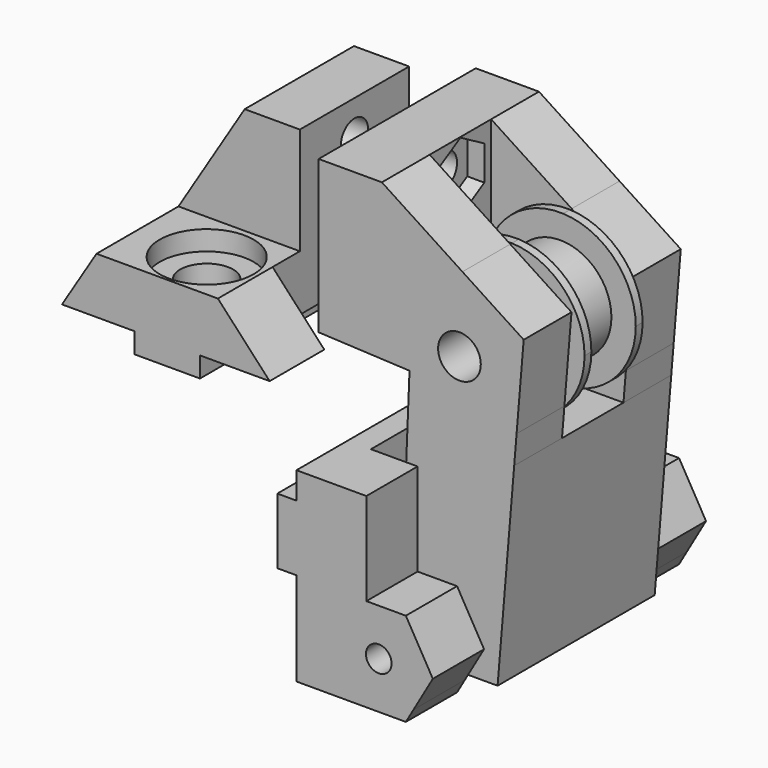
from build123d import *

# Parameters (mm, degrees)
F0_R      = 1.5
F1_DEPTH  = 20
F2_DEPTH  = 12.5
F0_R_2    = 6
F0_R_3    = 2.5
F3_DEPTH  = 4.25
F4_DEPTH  = 3.25
F5_DEPTH  = 11.5
F6_DEPTH  = 4.5
F7_DEPTH  = 20
F0_W      = 6.4631571341
F0_H      = 12.5490699407
F8_DEPTH  = 8
F9_DEPTH  = 5
F10_R     = 2
F11_DEPTH = 25
F12_DEPTH = 2
F13_R     = 3.1
F14_DEPTH = 9.6
F13_R_2   = 5.5
F15_DEPTH = 2.3
F16_DEPTH = 12


# Not quite as in the source:
# - a feature names something its author has since deleted; it is built from what else it names


with BuildPart() as f1:
    # F0 (on Front) → F1 (new body, symmetric)
    with BuildSketch(Plane.XZ):
        Polygon((12.0433680713, 8.4268744104), (9.800856933, 8.4268744104), (9.800856933, 0.7268744104), (12.0433680713, 0.7268744104), (12.0433680713, -4.5145147916), (12.0433680713, -4.9838108923), (12.0433680713, -10.2252000943), (14.7645920515, -10.2252000943), (14.7645920515, 11.5647632629), (12.0433680713, 11.5647632629), align=None)
        Polygon((18.1240398149, 11.5647632629), (14.7645920515, 11.5647632629), (14.7645920515, -10.2252000943), (24.8542597735, -10.2252000943), (25.7545311213, -8.6658843793), (17.3043143004, -8.6658843793), align=None)
        Polygon((20.2310747576, 11.5647632629), (18.1240398149, 11.5647632629), (17.3043143004, -8.6658843793), (25.7545311213, -8.6658843793), (28.0158513552, -4.749162842), (24.8542597735, 0.7268744104), (20.2310747576, 0.7268744104), align=None)
        with Locations((21.6832533479, -4.7491648653)):
            Circle(F0_R, mode=Mode.SUBTRACT)
    extrude(amount=F1_DEPTH, both=True)

    # F0 (on Front) → F2 (cut, symmetric)
    with BuildSketch(Plane.XZ):
        Polygon((20.2310747576, 11.5647632629), (18.1240398149, 11.5647632629), (17.3043143004, -8.6658843793), (25.7545311213, -8.6658843793), (28.0158513552, -4.749162842), (24.8542597735, 0.7268744104), (20.2310747576, 0.7268744104), align=None)
        with Locations((21.6832533479, -4.7491648653)):
            Circle(F0_R, mode=Mode.SUBTRACT)
        Polygon((18.1240398149, 11.5647632629), (14.7645920515, 11.5647632629), (14.7645920515, -10.2252000943), (24.8542597735, -10.2252000943), (25.7545311213, -8.6658843793), (17.3043143004, -8.6658843793), align=None)
    extrude(amount=F2_DEPTH, both=True, mode=Mode.SUBTRACT)


with BuildPart() as f3:
    # F0 (on Front) → F3 (new body, symmetric)
    with BuildSketch(Plane.XZ):
        with BuildLine():
            Line((18.4845160693, 20.4612389207), (18.3568896242, 17.3114459771))
            ThreePointArc((18.3568896242, 17.3114459771), (24.8470334947, 15.0024096492), (31.0266731703, 18.0463659077))
            Line((31.0266731703, 18.0463659077), (31.8562861888, 28.0017219973))
            Line((31.8562861888, 28.0017219973), (24.6849621756, 32.6806183183))
            ThreePointArc((24.6849621756, 32.6806183183), (17.1127643071, 28.953063684), (16.1086398476, 20.5730530528))
            Line((16.1086398476, 20.5730530528), (18.4845160693, 20.4612389207))
        make_face()
        with Locations((24.3345443159, 23.8375584789)):
            Circle(F0_R_2, mode=Mode.SUBTRACT)
        with Locations((24.3345443159, 23.8375584789)):
            Circle(F0_R_2)
        with Locations((24.3345443159, 23.8375584789)):
            Circle(F0_R_3, mode=Mode.SUBTRACT)
        with BuildLine():
            Line((31.8562861888, 28.0017219973), (31.0266731703, 18.0463659077))
            ThreePointArc((31.0266731703, 18.0463659077), (32.6275486075, 20.7474808392), (33.1845443159, 23.8375584789))
            ThreePointArc((33.1845443159, 23.8375584789), (30.7151280689, 29.970310795), (24.6849621756, 32.6806183183))
            Line((24.6849621756, 32.6806183183), (31.8562861888, 28.0017219973))
        make_face()
        with BuildLine():
            ThreePointArc((16.1086398476, 20.5730530528), (17.0479268988, 18.8148394327), (18.3568896242, 17.3114459771))
            Line((18.3568896242, 17.3114459771), (18.4845160693, 20.4612389207))
            Line((18.4845160693, 20.4612389207), (16.1086398476, 20.5730530528))
        make_face()
    extrude(amount=F3_DEPTH, both=True)

    # F0 (on Front) → F4 (cut, symmetric)
    with BuildSketch(Plane.XZ):
        with BuildLine():
            Line((31.8562861888, 28.0017219973), (31.0266731703, 18.0463659077))
            ThreePointArc((31.0266731703, 18.0463659077), (32.6275486075, 20.7474808392), (33.1845443159, 23.8375584789))
            ThreePointArc((33.1845443159, 23.8375584789), (30.7151280689, 29.970310795), (24.6849621756, 32.6806183183))
            Line((24.6849621756, 32.6806183183), (31.8562861888, 28.0017219973))
        make_face()
        with BuildLine():
            Line((18.4845160693, 20.4612389207), (18.3568896242, 17.3114459771))
            ThreePointArc((18.3568896242, 17.3114459771), (24.8470334947, 15.0024096492), (31.0266731703, 18.0463659077))
            Line((31.0266731703, 18.0463659077), (31.8562861888, 28.0017219973))
            Line((31.8562861888, 28.0017219973), (24.6849621756, 32.6806183183))
            ThreePointArc((24.6849621756, 32.6806183183), (17.1127643071, 28.953063684), (16.1086398476, 20.5730530528))
            Line((16.1086398476, 20.5730530528), (18.4845160693, 20.4612389207))
        make_face()
        with Locations((24.3345443159, 23.8375584789)):
            Circle(F0_R_2, mode=Mode.SUBTRACT)
        with BuildLine():
            ThreePointArc((16.1086398476, 20.5730530528), (17.0479268988, 18.8148394327), (18.3568896242, 17.3114459771))
            Line((18.3568896242, 17.3114459771), (18.4845160693, 20.4612389207))
            Line((18.4845160693, 20.4612389207), (16.1086398476, 20.5730530528))
        make_face()
    extrude(amount=F4_DEPTH, both=True, mode=Mode.SUBTRACT)


with BuildPart() as f5:
    # F0 (on Front) → F5 (new body, symmetric)
    with BuildSketch(Plane.XZ):
        with BuildLine():
            Line((18.4845160693, 20.4612389207), (18.3568896242, 17.3114459771))
            ThreePointArc((18.3568896242, 17.3114459771), (24.8470334947, 15.0024096492), (31.0266731703, 18.0463659077))
            Line((31.0266731703, 18.0463659077), (31.8562861888, 28.0017219973))
            Line((31.8562861888, 28.0017219973), (24.6849621756, 32.6806183183))
            ThreePointArc((24.6849621756, 32.6806183183), (17.1127643071, 28.953063684), (16.1086398476, 20.5730530528))
            Line((16.1086398476, 20.5730530528), (18.4845160693, 20.4612389207))
        make_face()
        with Locations((24.3345443159, 23.8375584789)):
            Circle(F0_R_2, mode=Mode.SUBTRACT)
        Polygon((18.2491015751, 14.6512603387), (18.1240398149, 11.5647632629), (20.2310747576, 11.5647632629), (20.2310747576, 0.7268744104), (24.8542597735, 0.7268744104), (28.0158513552, -4.749162842), (25.7545311213, -8.6658843793), (28.8006522836, -8.6658843793), (30.7437477025, 14.6512603387), align=None)
        Polygon((7.8407172114, 20.9621602735), (15.2479996905, 20.6135567336), (15.2479996905, 38.8377197087), (7.8407172114, 38.8377197087), align=None)
        with Locations((24.3345443159, 23.8375584789)):
            Circle(F0_R_2)
        with Locations((24.3345443159, 23.8375584789)):
            Circle(F0_R_3, mode=Mode.SUBTRACT)
        Polygon((20.2310747576, 11.5647632629), (18.1240398149, 11.5647632629), (17.3043143004, -8.6658843793), (25.7545311213, -8.6658843793), (28.0158513552, -4.749162842), (24.8542597735, 0.7268744104), (20.2310747576, 0.7268744104), align=None)
        with Locations((21.6832533479, -4.7491648653)):
            Circle(F0_R, mode=Mode.SUBTRACT)
        with BuildLine():
            Line((15.2479996905, 20.6135567336), (16.1086398476, 20.5730530528))
            ThreePointArc((16.1086398476, 20.5730530528), (17.1127643071, 28.953063684), (24.6849621756, 32.6806183183))
            Line((24.6849621756, 32.6806183183), (15.2479996905, 38.8377197087))
            Line((15.2479996905, 38.8377197087), (15.2479996905, 20.6135567336))
        make_face()
        with BuildLine():
            Line((18.3568896242, 17.3114459771), (18.2491015751, 14.6512603387))
            Line((18.2491015751, 14.6512603387), (30.7437477025, 14.6512603387))
            Line((30.7437477025, 14.6512603387), (31.0266731703, 18.0463659077))
            ThreePointArc((31.0266731703, 18.0463659077), (24.8470334947, 15.0024096492), (18.3568896242, 17.3114459771))
        make_face()
    extrude(amount=F5_DEPTH, both=True)

    # F0 (on Front) → F6 (cut, symmetric)
    with BuildSketch(Plane.XZ):
        with BuildLine():
            Line((18.4845160693, 20.4612389207), (18.3568896242, 17.3114459771))
            ThreePointArc((18.3568896242, 17.3114459771), (24.8470334947, 15.0024096492), (31.0266731703, 18.0463659077))
            Line((31.0266731703, 18.0463659077), (31.8562861888, 28.0017219973))
            Line((31.8562861888, 28.0017219973), (24.6849621756, 32.6806183183))
            ThreePointArc((24.6849621756, 32.6806183183), (17.1127643071, 28.953063684), (16.1086398476, 20.5730530528))
            Line((16.1086398476, 20.5730530528), (18.4845160693, 20.4612389207))
        make_face()
        with Locations((24.3345443159, 23.8375584789)):
            Circle(F0_R_2, mode=Mode.SUBTRACT)
        with Locations((24.3345443159, 23.8375584789)):
            Circle(F0_R_2)
        with Locations((24.3345443159, 23.8375584789)):
            Circle(F0_R_3, mode=Mode.SUBTRACT)
        with Locations((24.3345443159, 23.8375584789)):
            Circle(F0_R_3)
        with BuildLine():
            Line((18.3568896242, 17.3114459771), (18.2491015751, 14.6512603387))
            Line((18.2491015751, 14.6512603387), (30.7437477025, 14.6512603387))
            Line((30.7437477025, 14.6512603387), (31.0266731703, 18.0463659077))
            ThreePointArc((31.0266731703, 18.0463659077), (24.8470334947, 15.0024096492), (18.3568896242, 17.3114459771))
        make_face()
        with BuildLine():
            Line((15.2479996905, 20.6135567336), (16.1086398476, 20.5730530528))
            ThreePointArc((16.1086398476, 20.5730530528), (17.1127643071, 28.953063684), (24.6849621756, 32.6806183183))
            Line((24.6849621756, 32.6806183183), (15.2479996905, 38.8377197087))
            Line((15.2479996905, 38.8377197087), (15.2479996905, 20.6135567336))
        make_face()
    extrude(amount=F6_DEPTH, both=True, mode=Mode.SUBTRACT)


with BuildPart() as f7:
    # F0 (on Front) → F7 (new body, symmetric)
    with BuildSketch(Plane.XZ):
        Polygon((0.7433667779, 19.7268745396), (2.8407172114, 19.7268745396), (2.8407172114, 26.2715246085), (-3.6224399228, 26.2715246085), (-11.3784734885, 26.2715246085), (-15.4234366491, 19.7268745396), (-6.9566332221, 19.7268745396), (-6.9566332221, 17.3414862657), (0.7433667779, 17.3414862657), align=None)
        Polygon((2.8407172114, 26.2715246085), (2.8407172114, 19.7268745396), (8.9014992118, 19.7268745396), align=None)
    extrude(amount=F7_DEPTH, both=True)

    # F0 (on Front) → F8 (join, symmetric)
    with BuildSketch(Plane.XZ):
        with Locations((-0.3908613557, 32.5460595788)):
            Rectangle(F0_W, F0_H)
        Polygon((-11.3784734885, 26.2715246085), (-3.6224399228, 26.2715246085), (-3.6224399228, 38.8205945492), align=None)
    extrude(amount=F8_DEPTH, both=True)

    # F0 (on Front) → F9 (cut, symmetric)
    with BuildSketch(Plane.XZ):
        Polygon((-11.3784734885, 26.2715246085), (-3.6224399228, 26.2715246085), (-3.6224399228, 38.8205945492), align=None)
    extrude(amount=F9_DEPTH, both=True, mode=Mode.SUBTRACT)


with BuildPart() as f11_tool:
    # F10 (on face) → F11 (new body)
    with BuildSketch(Plane.YZ.offset(15.2479996905)):
        with Locations((0, 34.7265526652)):
            Circle(F10_R)
    extrude(amount=-F11_DEPTH)


with BuildPart() as f5_1:
    add(f5.part)

    # F11: cut by f11_tool
    add(f11_tool.part, mode=Mode.SUBTRACT)

    # F10 (on face) → F12 (cut)
    with BuildSketch(Plane.YZ.offset(15.2479996905)):
        Polygon((3.5, 36.7472786074), (0, 38.7680045496), (-3.5, 36.7472786074), (-3.5, 32.7058267231), (0, 30.6851007809), (3.5, 32.7058267231), align=None)
        with Locations((0, 34.7265526652)):
            Circle(F10_R, mode=Mode.SUBTRACT)
    extrude(amount=-F12_DEPTH, mode=Mode.SUBTRACT)


with BuildPart() as f7_1:
    add(f7.part)

    # F11: cut by f11_tool
    add(f11_tool.part, mode=Mode.SUBTRACT)

    # F13 (on face) → F14 (cut, symmetric)
    with BuildSketch(Plane.XY.offset(26.2715246085)):
        with Locations((-3.1142163277, 13.877896592)):
            Circle(F13_R)
        with Locations((-3.1142163277, -14.2000038177)):
            Circle(F13_R)
    extrude(amount=F14_DEPTH, both=True, mode=Mode.SUBTRACT)

    # F13 (on face) → F15 (cut, symmetric)
    with BuildSketch(Plane.XY.offset(26.2715246085)):
        with Locations((-3.1142163277, 13.877896592)):
            Circle(F13_R_2)
        with Locations((-3.1142163277, 13.877896592)):
            Circle(F13_R, mode=Mode.SUBTRACT)
        with Locations((-3.1142163277, -14.2000038177)):
            Circle(F13_R_2)
        with Locations((-3.1142163277, -14.2000038177)):
            Circle(F13_R, mode=Mode.SUBTRACT)
    extrude(amount=F15_DEPTH, both=True, mode=Mode.SUBTRACT)

    # F0 (on Front) → F16 (cut, symmetric)
    with BuildSketch(Plane.XZ):
        Polygon((2.8407172114, 26.2715246085), (2.8407172114, 19.7268745396), (8.9014992118, 19.7268745396), align=None)
    extrude(amount=F16_DEPTH, both=True, mode=Mode.SUBTRACT)


with BuildPart() as f17_1:
    # F17: copy of F3
    add(f3.part)


solid = Compound([f1.part, f3.part, f5_1.part, f7_1.part, f17_1.part])
